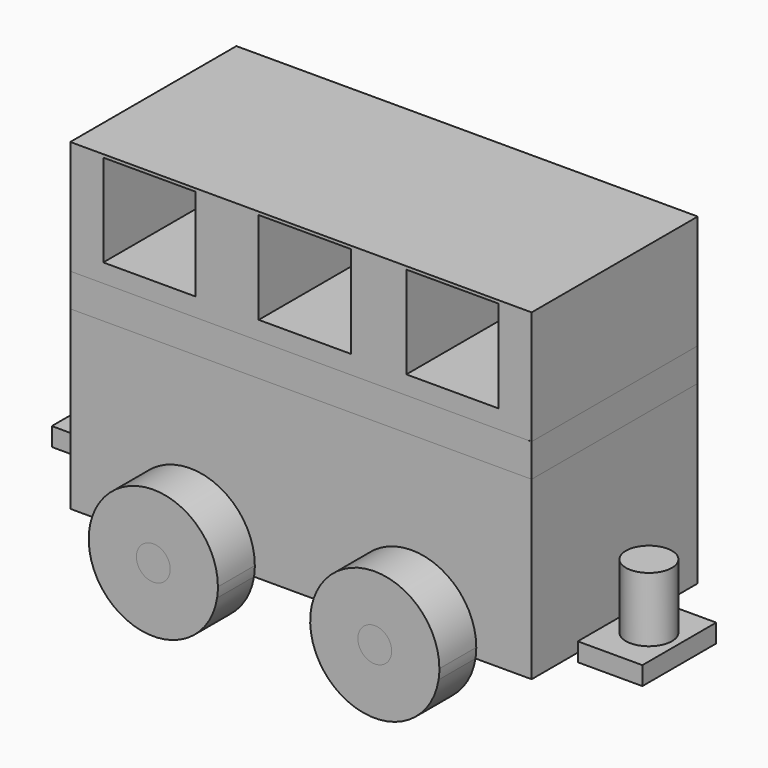
from build123d import *

# Parameters (mm, degrees)
F0_W          = 127
F0_H          = 31.3182
F0_W_2        = 25.4
F0_H_2        = 25.4
F1_DEPTH      = 28.575
F0_H_3        = 48.4632
F0_H_4        = 9.1186
F2_DEPTH      = 28.575
F4_DEPTH      = 12.7
F6_DEPTH      = 23.114
F7_DEPTH      = 82.804
F7_DEPTH_BACK = 76.2
F8_DEPTH      = 69.85
F8_DEPTH_BACK = 12.7
F9_W          = 25.4
F9_H          = 5.08
F10_DEPTH     = 17.78
F11_R         = 6.35
F12_DEPTH     = 17.78
F13_W         = 25.4
F13_H         = 5.08
F14_DEPTH     = 17.78
F15_R         = 6.35
F16_DEPTH     = 25.4


with BuildPart() as f1:
    # F0 (on Front) → F1 (new body, symmetric)
    with BuildSketch(Plane.XZ):
        with Locations((5.8995515195, 53.2792696041)):
            Rectangle(F0_W, F0_H)
        with Locations((-35.8146865249, 55.4001696041)):
            Rectangle(F0_W_2, F0_H_2, mode=Mode.SUBTRACT)
        with Locations((6.9737978751, 55.4001696041)):
            Rectangle(F0_W_2, F0_H_2, mode=Mode.SUBTRACT)
        with Locations((47.6137937195, 55.4001696041)):
            Rectangle(F0_W_2, F0_H_2, mode=Mode.SUBTRACT)
    extrude(amount=F1_DEPTH, both=True)

    # F3 (on face) → F6 (cut)
    with BuildSketch(Plane.XZ.offset(28.575)):
        with BuildLine():
            Line((-28.3030916435, -19.9616303959), (-42.1412203564, -19.9616303959))
            ThreePointArc((-42.1412203564, -19.9616303959), (-24.5804484805, -34.9581629324), (-7.0196766045, -19.9616303959))
            Line((-7.0196766045, -19.9616303959), (-20.8578053174, -19.9616303959))
            ThreePointArc((-20.8578053174, -19.9616303959), (-24.5804484805, -21.8263629324), (-28.3030916435, -19.9616303959))
        make_face()
        with BuildLine():
            Line((32.6569083565, -19.9616303959), (18.8187796436, -19.9616303959))
            ThreePointArc((18.8187796436, -19.9616303959), (36.3795515195, -34.9581629324), (53.9403233955, -19.9616303959))
            Line((53.9403233955, -19.9616303959), (40.1021946826, -19.9616303959))
            ThreePointArc((40.1021946826, -19.9616303959), (36.3795515195, -21.8263629324), (32.6569083565, -19.9616303959))
        make_face()
    extrude(amount=-F6_DEPTH, mode=Mode.SUBTRACT)


with BuildPart() as f1b:
    # F0 (on Front) → F1, piece 2 (new body, symmetric)
    with BuildSketch(Plane.XZ):
        with Locations((5.8995515195, 4.2699696041)):
            Rectangle(F0_W, F0_H_3)
    extrude(amount=F1_DEPTH, both=True)

    # F3 (on face) → F7 (cut, two sides)
    with BuildSketch(Plane.XZ.offset(28.575)) as f7_sk:
        with BuildLine():
            Line((40.1021946826, -19.9616303959), (32.6569083565, -19.9616303959))
            ThreePointArc((32.6569083565, -19.9616303959), (36.3795515195, -21.8263629324), (40.1021946826, -19.9616303959))
        make_face()
        with BuildLine():
            ThreePointArc((41.0277515195, -17.1781629324), (34.9128931937, -12.7674173497), (32.6569083565, -19.9616303959))
            Line((32.6569083565, -19.9616303959), (40.1021946826, -19.9616303959))
            ThreePointArc((40.1021946826, -19.9616303959), (40.7902971022, -18.6448212582), (41.0277515195, -17.1781629324))
        make_face()
        with BuildLine():
            Line((-20.8578053174, -19.9616303959), (-28.3030916435, -19.9616303959))
            ThreePointArc((-28.3030916435, -19.9616303959), (-24.5804484805, -21.8263629324), (-20.8578053174, -19.9616303959))
        make_face()
        with BuildLine():
            ThreePointArc((-19.9322484805, -17.1781629324), (-26.0471068063, -12.7674173497), (-28.3030916435, -19.9616303959))
            Line((-28.3030916435, -19.9616303959), (-20.8578053174, -19.9616303959))
            ThreePointArc((-20.8578053174, -19.9616303959), (-20.1697028978, -18.6448212582), (-19.9322484805, -17.1781629324))
        make_face()
    extrude(amount=-F7_DEPTH, mode=Mode.SUBTRACT)
    extrude(f7_sk.sketch, amount=F7_DEPTH_BACK, mode=Mode.SUBTRACT)

    # F9 (on face) → F10 (join)
    with BuildSketch(Plane.YZ.offset(69.3995515195)):
        with Locations((0, -19.7584303959)):
            Rectangle(F9_W, F9_H)
    extrude(amount=F10_DEPTH)

    # F11 (on face) → F12 (join)
    with BuildSketch(Plane.XY.offset(-17.2184303959)):
        with Locations((78.8229515195, 0)):
            Circle(F11_R)
    extrude(amount=F12_DEPTH)

    # F13 (on face) → F14 (join)
    with BuildSketch(Plane(origin=(-57.6004484805, 0, 0), x_dir=(0, -1, 0), z_dir=(-1, 0, 0))):
        with Locations((0, -14.6784303959)):
            Rectangle(F13_W, F13_H)
    extrude(amount=F14_DEPTH)

    # F15 (on face) → F16 (cut)
    with BuildSketch(Plane.XY.offset(-12.1384303959)):
        with Locations((-67.0238484805, 0)):
            Circle(F15_R)
    extrude(amount=-F16_DEPTH, mode=Mode.SUBTRACT)


with BuildPart() as f2:
    # F0 (on Front) → F2 (new body, symmetric)
    with BuildSketch(Plane.XZ):
        with Locations((5.8995515195, 33.0608696041)):
            Rectangle(F0_W, F0_H_4)
    extrude(amount=F2_DEPTH, both=True)


with BuildPart() as f4:
    # F3 (on face) → F4 (new body)
    with BuildSketch(Plane.XZ.offset(28.575)):
        with BuildLine():
            Line((-28.3030916435, -19.9616303959), (-42.1412203564, -19.9616303959))
            ThreePointArc((-42.1412203564, -19.9616303959), (-24.5804484805, -34.9581629324), (-7.0196766045, -19.9616303959))
            Line((-7.0196766045, -19.9616303959), (-20.8578053174, -19.9616303959))
            ThreePointArc((-20.8578053174, -19.9616303959), (-24.5804484805, -21.8263629324), (-28.3030916435, -19.9616303959))
        make_face()
        with BuildLine():
            ThreePointArc((-7.0196766045, -19.9616303959), (-6.8553402445, -18.5742066361), (-6.8004484805, -17.1781629324))
            ThreePointArc((-6.8004484805, -17.1781629324), (-25.9764921842, 0.5469453036), (-42.1412203564, -19.9616303959))
            Line((-42.1412203564, -19.9616303959), (-28.3030916435, -19.9616303959))
            ThreePointArc((-28.3030916435, -19.9616303959), (-26.0471068063, -12.7674173497), (-19.9322484805, -17.1781629324))
            ThreePointArc((-19.9322484805, -17.1781629324), (-20.1697028978, -18.6448212582), (-20.8578053174, -19.9616303959))
            Line((-20.8578053174, -19.9616303959), (-7.0196766045, -19.9616303959))
        make_face()
    extrude(amount=F4_DEPTH)


with BuildPart() as f4b:
    # F3 (on face) → F4, piece 2 (new body)
    with BuildSketch(Plane.XZ.offset(28.575)):
        with BuildLine():
            Line((32.6569083565, -19.9616303959), (18.8187796436, -19.9616303959))
            ThreePointArc((18.8187796436, -19.9616303959), (36.3795515195, -34.9581629324), (53.9403233955, -19.9616303959))
            Line((53.9403233955, -19.9616303959), (40.1021946826, -19.9616303959))
            ThreePointArc((40.1021946826, -19.9616303959), (36.3795515195, -21.8263629324), (32.6569083565, -19.9616303959))
        make_face()
        with BuildLine():
            ThreePointArc((54.1595515195, -17.1781629324), (34.9835078158, 0.5469453036), (18.8187796436, -19.9616303959))
            Line((18.8187796436, -19.9616303959), (32.6569083565, -19.9616303959))
            ThreePointArc((32.6569083565, -19.9616303959), (34.9128931937, -12.7674173497), (41.0277515195, -17.1781629324))
            ThreePointArc((41.0277515195, -17.1781629324), (40.7902971022, -18.6448212582), (40.1021946826, -19.9616303959))
            Line((40.1021946826, -19.9616303959), (53.9403233955, -19.9616303959))
            ThreePointArc((53.9403233955, -19.9616303959), (54.1046597555, -18.5742066361), (54.1595515195, -17.1781629324))
        make_face()
    extrude(amount=F4_DEPTH)


with BuildPart() as f5_1:
    # F5: instance of F4
    add(f4.part.mirror(Plane.XZ))


with BuildPart() as f5_2:
    # F5: instance of F4b
    add(f4b.part.mirror(Plane.XZ))


with BuildPart() as f8:
    # F3 (on face) → F8 (new body, two sides)
    with BuildSketch(Plane.XZ.offset(28.575)) as f8_sk:
        with BuildLine():
            Line((-20.8578053174, -19.9616303959), (-28.3030916435, -19.9616303959))
            ThreePointArc((-28.3030916435, -19.9616303959), (-24.5804484805, -21.8263629324), (-20.8578053174, -19.9616303959))
        make_face()
        with BuildLine():
            ThreePointArc((-19.9322484805, -17.1781629324), (-26.0471068063, -12.7674173497), (-28.3030916435, -19.9616303959))
            Line((-28.3030916435, -19.9616303959), (-20.8578053174, -19.9616303959))
            ThreePointArc((-20.8578053174, -19.9616303959), (-20.1697028978, -18.6448212582), (-19.9322484805, -17.1781629324))
        make_face()
    extrude(amount=-F8_DEPTH)
    extrude(f8_sk.sketch, amount=F8_DEPTH_BACK)


with BuildPart() as f8b:
    # F3 (on face) → F8, piece 2 (new body, two sides)
    with BuildSketch(Plane.XZ.offset(28.575)) as f8_2_sk:
        with BuildLine():
            Line((40.1021946826, -19.9616303959), (32.6569083565, -19.9616303959))
            ThreePointArc((32.6569083565, -19.9616303959), (36.3795515195, -21.8263629324), (40.1021946826, -19.9616303959))
        make_face()
        with BuildLine():
            ThreePointArc((41.0277515195, -17.1781629324), (34.9128931937, -12.7674173497), (32.6569083565, -19.9616303959))
            Line((32.6569083565, -19.9616303959), (40.1021946826, -19.9616303959))
            ThreePointArc((40.1021946826, -19.9616303959), (40.7902971022, -18.6448212582), (41.0277515195, -17.1781629324))
        make_face()
    extrude(amount=-F8_DEPTH)
    extrude(f8_2_sk.sketch, amount=F8_DEPTH_BACK)


solid = Compound([f1.part, f1b.part, f2.part, f4.part, f4b.part, f5_1.part, f5_2.part, f8.part, f8b.part])
